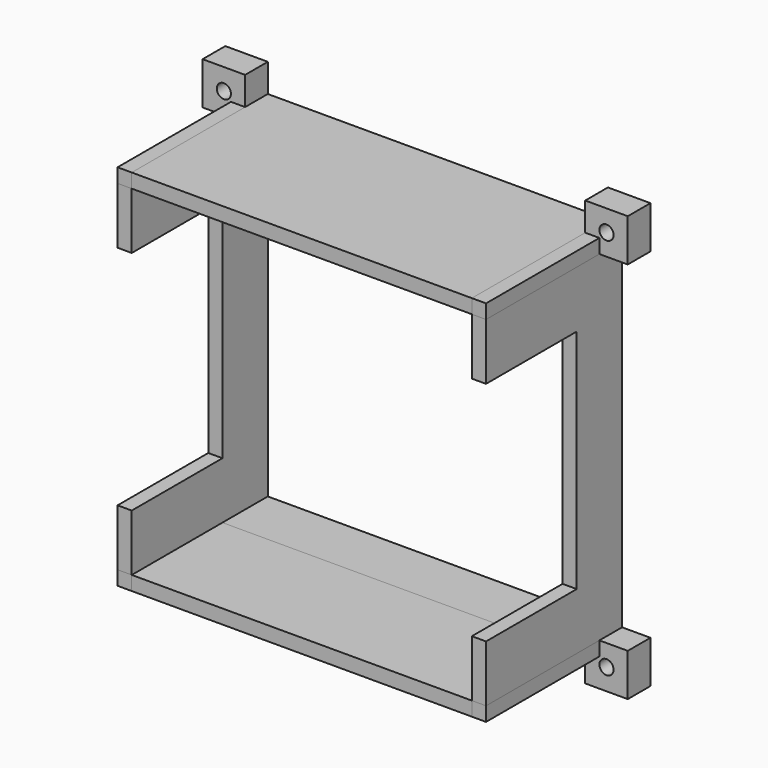
from build123d import *

# Parameters (mm, degrees)
F0_W     = 152.4
F0_H     = 6.35
F1_DEPTH = 76.2
F0_W_2   = 6.35
F0_H_2   = 152.4
F2_DEPTH = 25.4
F3_W     = 50.8
F3_H     = 101.6
F4_DEPTH = 254
F0_R     = 3.175
F5_DEPTH = 12.7
F6_DEPTH = 76.2
F7_DEPTH = 12.7


with BuildPart() as f1:
    # F0 (on Front) → F1 (new body)
    with BuildSketch(Plane.XZ):
        with Locations((0, 79.375)):
            Rectangle(F0_W, F0_H)
    extrude(amount=F1_DEPTH)

    # F0 (on Front) → F7 (cut)
    with BuildSketch(Plane.XZ):
        with Locations((85.725, 85.725)):
            Circle(F0_R)
        with Locations((-85.725, 85.725)):
            Circle(F0_R)
        Polygon((-82.55, -82.55), (-82.55, -76.2), (-95.25, -76.2), (-95.25, -95.25), (-76.2, -95.25), (-76.2, -82.55), align=None)
        with Locations((-85.725, -85.725)):
            Circle(F0_R, mode=Mode.SUBTRACT)
        with Locations((85.725, -85.725)):
            Circle(F0_R)
    extrude(amount=-F7_DEPTH, mode=Mode.SUBTRACT)


with BuildPart() as f1b:
    # F0 (on Front) → F1, piece 2 (new body)
    with BuildSketch(Plane.XZ):
        with Locations((-79.375, 0)):
            Rectangle(F0_W_2, F0_H_2)
    extrude(amount=F1_DEPTH)

    # F0 (on Front) → F2 (join)
    with BuildSketch(Plane.XZ):
        with Locations((0, -79.375)):
            Rectangle(F0_W, F0_H)
    extrude(amount=F2_DEPTH)


with BuildPart() as f1c:
    # F0 (on Front) → F1, piece 3 (new body)
    with BuildSketch(Plane.XZ):
        with Locations((79.375, 0)):
            Rectangle(F0_W_2, F0_H_2)
    extrude(amount=F1_DEPTH)


with BuildPart() as f1d:
    # F0 (on Front) → F1, piece 4 (new body)
    with BuildSketch(Plane.XZ):
        with Locations((0, -79.375)):
            Rectangle(F0_W, F0_H)
    extrude(amount=F1_DEPTH)


with BuildPart() as f4_tool:
    # F3 (on face) → F4 (new body)
    with BuildSketch(Plane.YZ.offset(82.55)):
        with Locations((-50.8, 0)):
            Rectangle(F3_W, F3_H)
    extrude(amount=-F4_DEPTH)


with BuildPart() as f1b_1:
    add(f1b.part)

    # F4: cut by f4_tool
    add(f4_tool.part, mode=Mode.SUBTRACT)


with BuildPart() as f1c_1:
    add(f1c.part)

    # F4: cut by f4_tool
    add(f4_tool.part, mode=Mode.SUBTRACT)


with BuildPart() as f5:
    # F0 (on Front) → F5 (new body)
    with BuildSketch(Plane.XZ):
        Polygon((-95.25, 76.2), (-82.55, 76.2), (-82.55, 82.55), (-76.2, 82.55), (-76.2, 95.25), (-95.25, 95.25), align=None)
        with Locations((-85.725, 85.725)):
            Circle(F0_R, mode=Mode.SUBTRACT)
    extrude(amount=F5_DEPTH)


with BuildPart() as f5b:
    # F0 (on Front) → F5, piece 2 (new body)
    with BuildSketch(Plane.XZ):
        Polygon((82.55, 82.55), (82.55, 76.2), (95.25, 76.2), (95.25, 95.25), (76.2, 95.25), (76.2, 82.55), align=None)
        with Locations((85.725, 85.725)):
            Circle(F0_R, mode=Mode.SUBTRACT)
    extrude(amount=F5_DEPTH)


with BuildPart() as f5c:
    # F0 (on Front) → F5, piece 3 (new body)
    with BuildSketch(Plane.XZ):
        Polygon((82.55, -82.55), (76.2, -82.55), (76.2, -95.25), (95.25, -95.25), (95.25, -76.2), (82.55, -76.2), align=None)
        with Locations((85.725, -85.725)):
            Circle(F0_R, mode=Mode.SUBTRACT)
    extrude(amount=F5_DEPTH)


with BuildPart() as f5d:
    # F0 (on Front) → F5, piece 4 (new body)
    with BuildSketch(Plane.XZ):
        Polygon((-82.55, -82.55), (-82.55, -76.2), (-95.25, -76.2), (-95.25, -95.25), (-76.2, -95.25), (-76.2, -82.55), align=None)
        with Locations((-85.725, -85.725)):
            Circle(F0_R, mode=Mode.SUBTRACT)
    extrude(amount=F5_DEPTH)


with BuildPart() as f6:
    # F0 (on Front) → F6 (new body)
    with BuildSketch(Plane.XZ):
        with Locations((-79.375, 79.375)):
            Rectangle(F0_W_2, F0_H)
    extrude(amount=F6_DEPTH)


with BuildPart() as f6b:
    # F0 (on Front) → F6, piece 2 (new body)
    with BuildSketch(Plane.XZ):
        with Locations((79.375, 79.375)):
            Rectangle(F0_W_2, F0_H)
    extrude(amount=F6_DEPTH)


with BuildPart() as f6c:
    # F0 (on Front) → F6, piece 3 (new body)
    with BuildSketch(Plane.XZ):
        with Locations((-79.375, -79.375)):
            Rectangle(F0_W_2, F0_H)
    extrude(amount=F6_DEPTH)


with BuildPart() as f6d:
    # F0 (on Front) → F6, piece 4 (new body)
    with BuildSketch(Plane.XZ):
        with Locations((79.375, -79.375)):
            Rectangle(F0_W_2, F0_H)
    extrude(amount=F6_DEPTH)


solid = Compound([f1.part, f1d.part, f1b_1.part, f1c_1.part, f5.part, f5b.part, f5c.part, f5d.part, f6.part, f6b.part, f6c.part, f6d.part])
